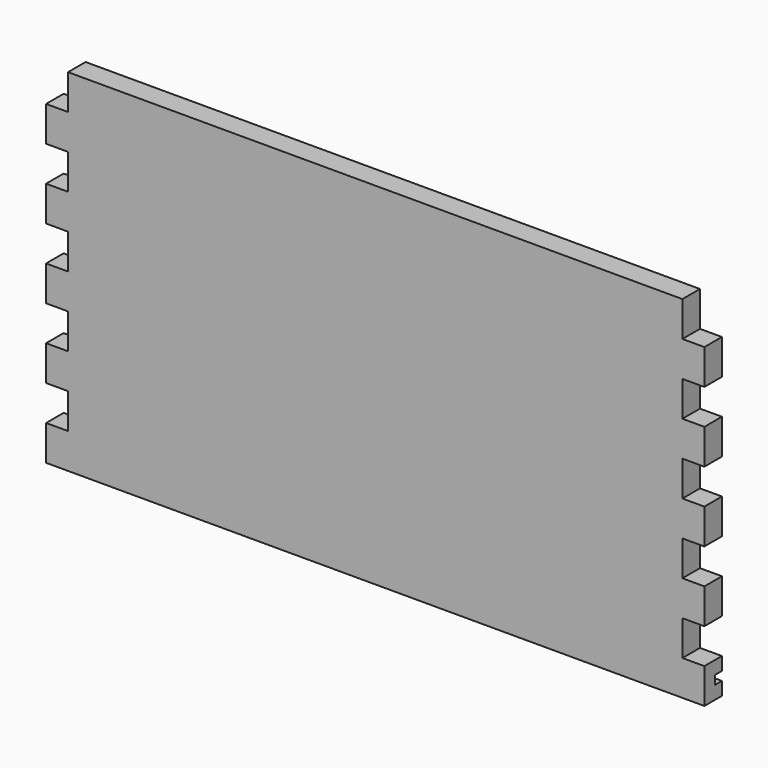
from build123d import *

# Parameters (mm, degrees)
F2_DEPTH = 5
F3_W     = 2
F3_H     = 2
F4_DEPTH = 150.001


# Not quite as in the source:
# - a feature names something its author has since deleted; it is built from what else it names


with BuildPart() as f2:
    # F1 (on Front) → F2 (new body)
    with BuildSketch(Plane.XZ):
        Polygon((70, -8), (70, 0), (-70, 0), (-70, -8), (-75, -8), (-75, -16), (-70, -16), (-70, -24), (-75, -24), (-75, -32), (-70, -32), (-70, -40), (-75, -40), (-75, -48), (-70, -48), (-70, -56), (-75, -56), (-75, -64), (-70, -64), (-70, -72), (-75, -72), (-75, -80), (75, -80), (75, -72), (70, -72), (70, -64), (75, -64), (75, -56), (70, -56), (70, -48), (75, -48), (75, -40), (70, -40), (70, -32), (75, -32), (75, -24), (70, -24), (70, -16), (75, -16), (75, -8), align=None)
    extrude(amount=F2_DEPTH)

    # F3 (on face) → F4 (cut, through all)
    with BuildSketch(Plane.YZ.offset(75)):
        with Locations((-1, -76)):
            Rectangle(F3_W, F3_H)
    extrude(amount=-F4_DEPTH, mode=Mode.SUBTRACT)


solid = f2.part
